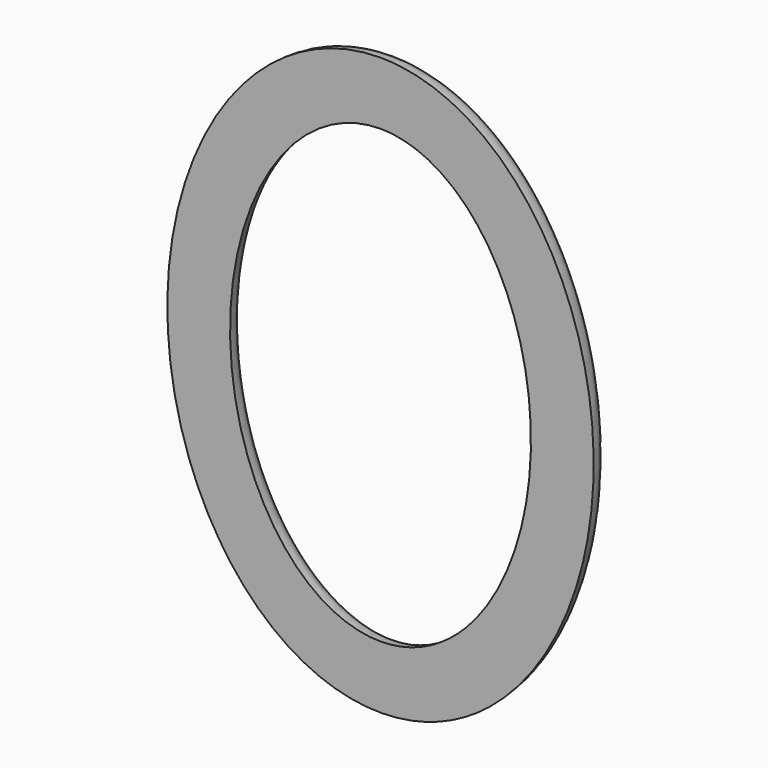
from build123d import *

# Parameters (mm, degrees)
F1_DEPTH = 25.4
F2_R     = 25.399
F3_R     = 25.399


# Not quite as in the source:
# - a fillet or chamfer is up to 0.001 mm smaller than in the source, because OpenCascade refuses the exact size


with BuildPart() as f1:
    # F0 (on Front) → F1 (new body)
    with BuildSketch(Plane.XZ):
        with BuildLine():
            add(Edge.make_bspline(
                [(0, 292.1), (-373.9497693541, 292.1), (-186.9748846771, -146.05), (0, -584.2), (186.9748846771, -146.05), (373.9497693541, 292.1), (0, 292.1)],
                knots=[0, 0, 0, 2.0943951024, 2.0943951024, 4.1887902048, 4.1887902048, 6.2831853072, 6.2831853072, 6.2831853072], degree=2, weights=[1, 0.5, 1, 0.5, 1, 0.5, 1]))
        make_face()
        with BuildLine():
            add(Edge.make_bspline(
                [(0, 228.6), (-263.9645430735, 228.6), (-131.9822715367, -114.3), (0, -457.2), (131.9822715367, -114.3), (263.9645430735, 228.6), (0, 228.6)],
                knots=[0, 0, 0, 2.0943951024, 2.0943951024, 4.1887902048, 4.1887902048, 6.2831853072, 6.2831853072, 6.2831853072], degree=2, weights=[1, 0.5, 1, 0.5, 1, 0.5, 1]))
        make_face(mode=Mode.SUBTRACT)
    extrude(amount=-F1_DEPTH)

    # F2 (radius 25.4 in the source; OpenCascade refuses exactly that, so slightly less here)
    f2_edges = [f1.edges().sort_by_distance(p)[0] for p in [
        (0, 25.4, -228.6),
    ]]
    fillet(f2_edges, radius=F2_R)

    # F3 (radius 25.4 in the source; OpenCascade refuses exactly that, so slightly less here)
    f3_edges = [f1.edges().sort_by_distance(p)[0] for p in [
        (0, 25.4, -292.1),
    ]]
    fillet(f3_edges, radius=F3_R)


solid = f1.part
